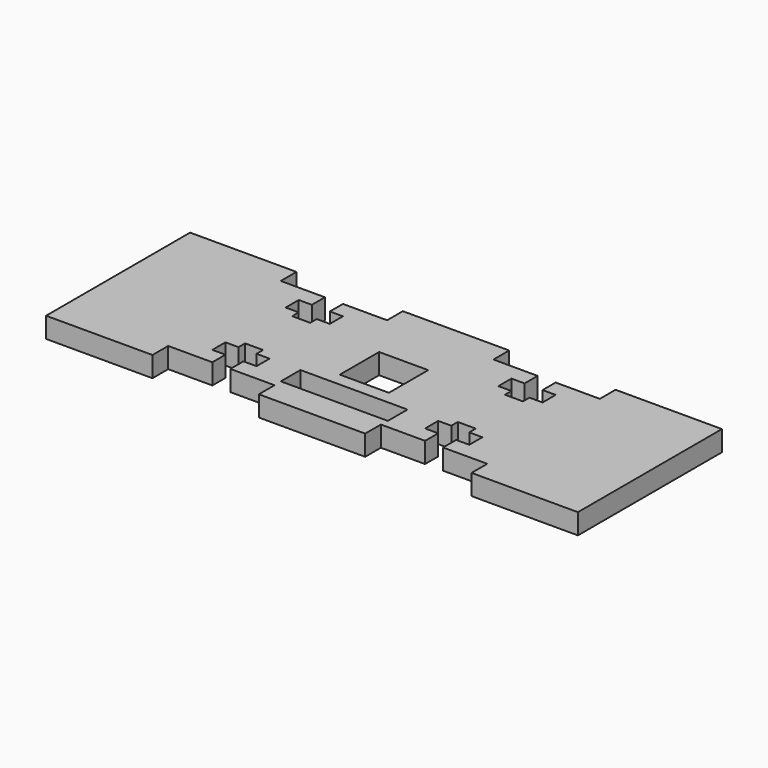
from build123d import *

# Parameters (mm, degrees)
F0_W     = 16.6126135737
F0_H     = 3.81
F0_W_2   = 7.62
F0_H_2   = 7.62
F1_DEPTH = 3.175


# Not quite as in the source:
# - a length typed as a fraction of an inch, garbled in the dataset ("3 / 203.2 mm" for 3/8 in), is restored
# - a feature names something its author has since deleted; it is built from what else it names


with BuildPart() as f1:
    # F0 (on Top) → F1 (new body)
    with BuildSketch(Plane.XY):
        Polygon((24.765, -8.001), (41.275, -8.001), (41.275, 19.939), (24.765, 19.939), (24.765, 16.891), (17.907, 16.891), (17.907, 14.351), (19.939, 14.351), (19.939, 11.811), (17.907, 11.811), (17.907, 10.541), (15.113, 10.541), (15.113, 11.811), (13.081, 11.811), (13.081, 14.351), (15.113, 14.351), (15.113, 16.891), (8.255, 16.891), (8.255, 19.939), (-8.255, 19.939), (-8.255, 16.891), (-15.113, 16.891), (-15.113, 14.351), (-13.081, 14.351), (-13.081, 11.811), (-15.113, 11.811), (-15.113, 10.541), (-17.907, 10.541), (-17.907, 11.811), (-19.939, 11.811), (-19.939, 14.351), (-17.907, 14.351), (-17.907, 16.891), (-24.765, 16.891), (-24.765, 19.939), (-41.275, 19.939), (-41.275, -8.001), (-24.765, -8.001), (-24.765, -4.953), (-17.907, -4.953), (-17.907, -2.413), (-19.939, -2.413), (-19.939, 0.127), (-17.907, 0.127), (-17.907, 1.397), (-15.113, 1.397), (-15.113, 0.127), (-13.081, 0.127), (-13.081, -2.413), (-15.113, -2.413), (-15.113, -4.953), (-8.255, -4.953), (-8.255, -8.001), (8.255, -8.001), (8.255, -4.953), (15.113, -4.953), (15.113, -2.413), (13.081, -2.413), (13.081, 0.127), (15.113, 0.127), (15.113, 1.397), (17.907, 1.397), (17.907, 0.127), (19.939, 0.127), (19.939, -2.413), (17.907, -2.413), (17.907, -4.953), (24.765, -4.953), align=None)
        with Locations((0.0095833093, -1.778)):
            Rectangle(F0_W, F0_H, mode=Mode.SUBTRACT)
        with Locations((0, 5.969)):
            Rectangle(F0_W_2, F0_H_2, mode=Mode.SUBTRACT)
    extrude(amount=F1_DEPTH)


solid = f1.part
